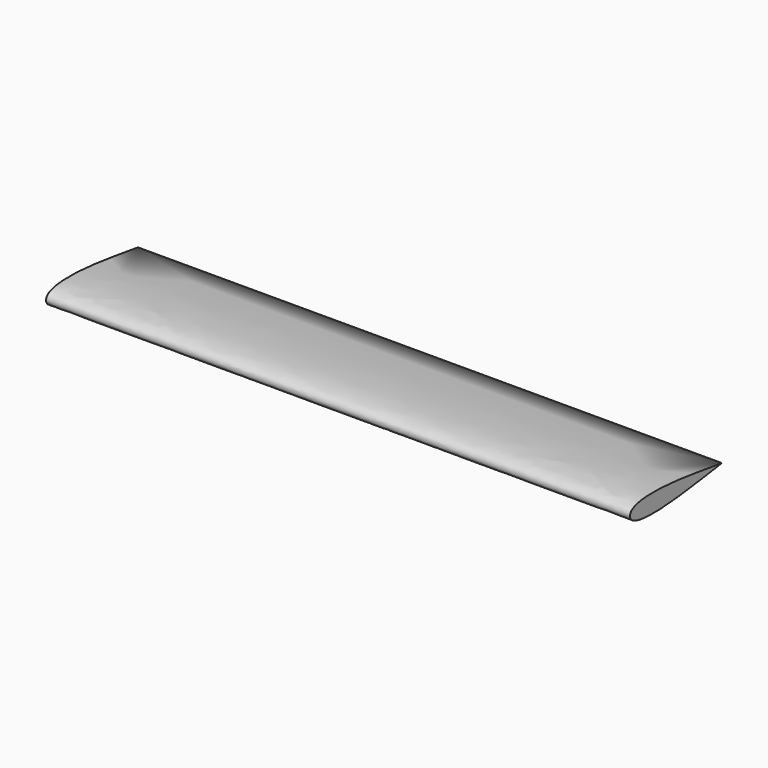
from build123d import *

# Parameters (mm, degrees)
F1_DEPTH = 508


with BuildPart() as f1:
    # F0 (on Right) → F1 (new body)
    with BuildSketch(Plane.YZ):
        with BuildLine():
            add(Edge.make_bspline(
                [(-48.2674092054, 0), (-48.2674092054, 5.9750759974), (-18.9687694723, 11.0118121173), (23.4132478852, 3.9461736604), (51.6283921897, 0)],
                knots=[0, 0, 0, 0, 0.357096586, 1, 1, 1, 1], degree=3))
            add(Edge.make_bspline(
                [(-48.2674092054, 0), (-48.2674092054, -5.9750759974), (-18.9687694723, -11.0118121173), (23.4132478852, -3.9461736604), (51.6283921897, 0)],
                knots=[0, 0, 0, 0, 0.357096586, 1, 1, 1, 1], degree=3))
        make_face()
    extrude(amount=F1_DEPTH)


solid = f1.part
